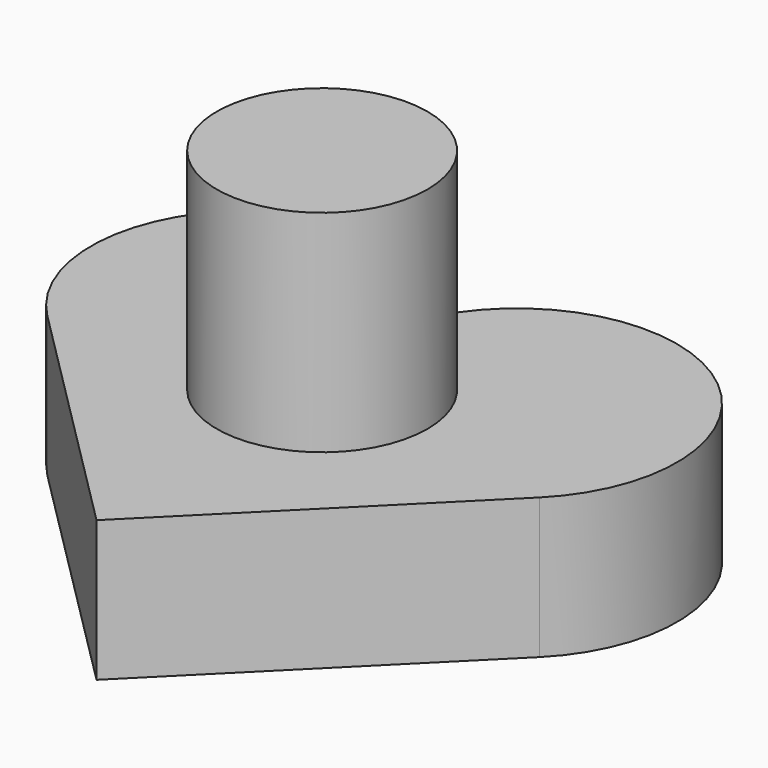
from build123d import *

# Parameters (mm, degrees)
F1_DEPTH     = 10
F2_R         = 7.5
F3_DEPTH     = 15
F4_TEXT_SIZE = 25
F5_DEPTH     = 4


# Not quite as in the source:
# - Text() gives the source's letters only with a copy of the font that has no kerning and outlines rounded to 1/6400 em; it was checked with that copy


with BuildPart() as f1:
    # F0 (on Top) → F1 (new body)
    with BuildSketch(Plane.XY):
        with BuildLine():
            Line((-17.5, 17.5), (0, 0))
            Line((0, 0), (17.5, 17.5))
            ThreePointArc((17.5, 17.5), (16.7114781519, 34.3586805281), (0, 32))
            ThreePointArc((0, 32), (-16.7114781519, 34.3586805281), (-17.5, 17.5))
        make_face()
    extrude(amount=F1_DEPTH)

    # F2 (on face) → F3 (join)
    with BuildSketch(Plane.XY.offset(10)):
        with Locations((0, 20.0624582583)):
            Circle(F2_R)
    extrude(amount=F3_DEPTH)

    # F4 (on Top) → F5 (cut)
    with BuildSketch(Plane.XY):
        with Locations((-9.716796875, 12)):
            Text('A', F4_TEXT_SIZE, font='Tinos', font_style=FontStyle.BOLD, text_align=(TextAlign.LEFT, TextAlign.BOTTOM))
    extrude(amount=F5_DEPTH, mode=Mode.SUBTRACT)


solid = f1.part
